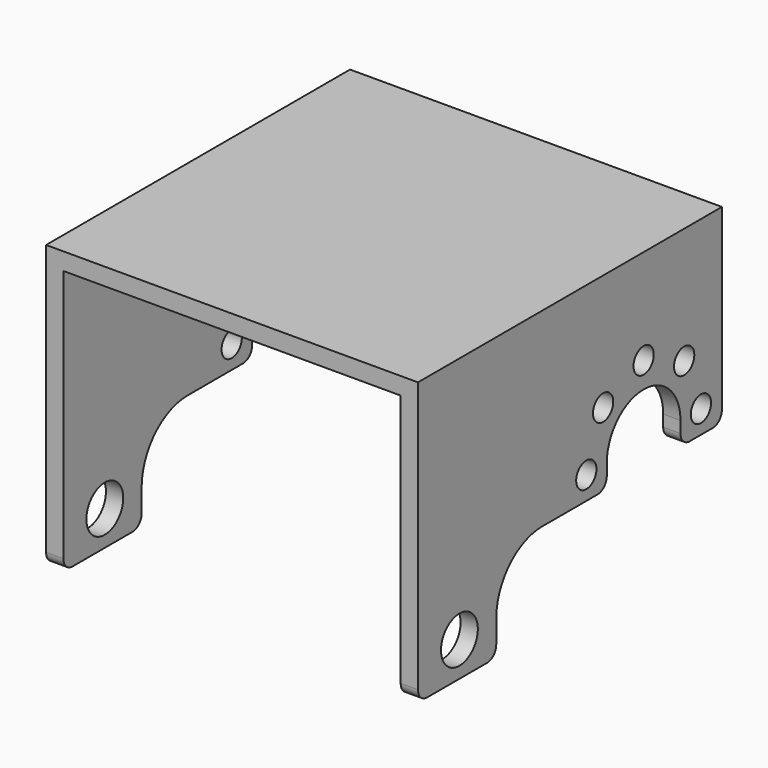
from build123d import *

# Parameters (mm, degrees)
F1_DEPTH = 33
F2_R     = 1.1
F2_R_2   = 2
F3_DEPTH = 32.301
F4_R     = 1
F5_R     = 5


with BuildPart() as f1:
    # F0 (on Front) → F1 (new body)
    with BuildSketch(Plane.XZ):
        Polygon((0, 24.5), (0, 0), (1.5, 0), (1.5, 23), (30.8, 23), (30.8, 0), (32.3, 0), (32.3, 24.5), align=None)
    extrude(amount=F1_DEPTH)

    # F2 (on face) → F3 (cut, through all)
    with BuildSketch(Plane(origin=(0, 0, 0), x_dir=(0, -1, 0), z_dir=(-1, 0, 0))):
        with BuildLine():
            Line((0, 8), (0, 0))
            Line((0, 0), (24.5, 0))
            Line((24.5, 0), (24.5, 8))
            Line((24.5, 8), (12.5, 8))
            Line((12.5, 8), (12.5, 10))
            ThreePointArc((12.5, 10), (8.5, 14), (4.5, 10))
            Line((4.5, 10), (4.5, 8))
            Line((4.5, 8), (0, 8))
        make_face()
        with Locations((14.7225396744, 10)):
            Circle(F2_R)
        with Locations((12.9, 14.4)):
            Circle(F2_R)
        with Locations((8.5, 16.2225396744)):
            Circle(F2_R)
        with Locations((4.1, 14.4)):
            Circle(F2_R)
        with Locations((2.2774603256, 10)):
            Circle(F2_R)
        with Locations((28.5, 3)):
            Circle(F2_R_2)
    extrude(amount=-F3_DEPTH, mode=Mode.SUBTRACT)

    # F4
    f4_edges = [f1.edges().sort_by_distance(p)[0] for p in [
        (0.75, -4.5, 8),
        (31.55, -4.5, 8),
        (0.75, -12.5, 8),
        (31.55, -12.5, 8),
        (31.55, 0, 8),
        (0.75, 0, 8),
        (0.75, -24.5, 0),
        (31.55, -24.5, 0),
        (0.75, -33, 0),
        (31.55, -33, 0),
    ]]
    fillet(f4_edges, radius=F4_R)

    # F5
    f5_edges = [f1.edges().sort_by_distance(p)[0] for p in [
        (0.75, -24.5, 8),
        (31.55, -24.5, 8),
    ]]
    fillet(f5_edges, radius=F5_R)


solid = f1.part
